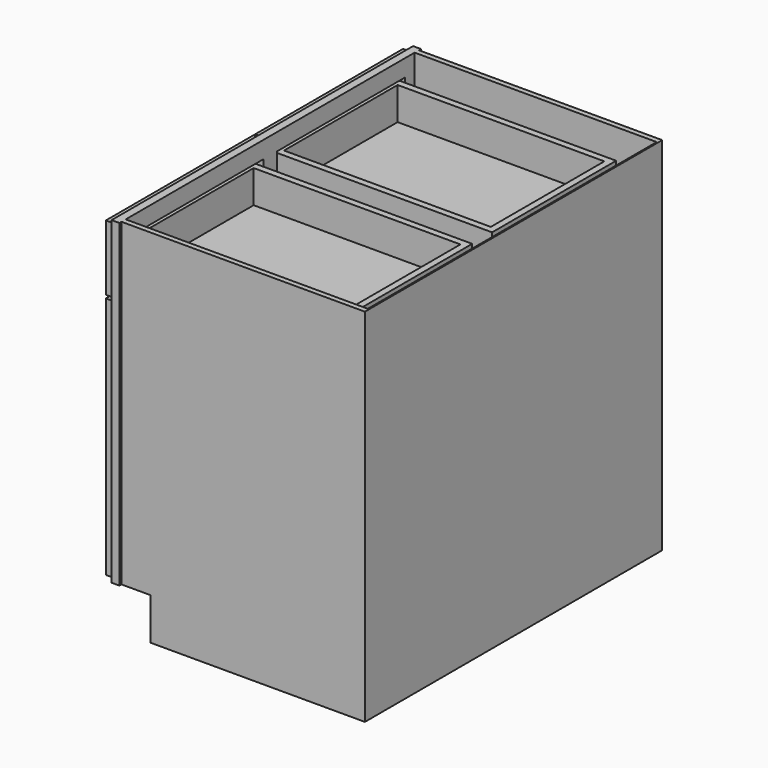
from build123d import *

# Parameters (mm, degrees)
F0_W          = 609.6
F0_H          = 876.3
F1_DEPTH      = 914.4
F2_W          = 88.9
F2_H          = 101.6
F3_DEPTH      = 914.401
F4_W          = 816.9639344262
F4_H          = 692.15
F5_DEPTH      = 19.05
F6_W          = 590.55
F6_H          = 6.35
F7_DEPTH      = 876.301
F8_W          = 587.375
F8_H          = 876.3
F9_DEPTH      = 733.425
F10_W         = 387.8444672131
F10_H         = 41.275
F10_W_2       = 41.275
F10_H_2       = 111.125
F10_H_3       = 539.75
F11_DEPTH     = 19.05
F12_W         = 448.46875
F12_H         = 590.5627
F12_W_2       = 334.16875
F12_H_2       = 476.2627
F13_DEPTH     = 19.05
F14_W         = 6.35
F14_H         = 334.16875
F15_DEPTH     = 476.2627
F16_SIZE      = 3.175
F17_W         = 448.46875
F17_H         = 158.75
F17_W_2       = 334.16875
F17_H_2       = 82.55
F18_DEPTH     = 19.05
F19_W         = 6.35
F19_H         = 334.16875
F20_DEPTH     = 82.55
F21_SIZE      = 3.175
F22_W         = 504.825
F22_H         = 876.3
F23_DEPTH     = 101.6
F24_W         = 376.2375
F24_H         = 95.25
F25_DEPTH     = 533.4
F26_T         = 15.875
F26_T3_DEPTH  = 37.249261314
F26_T5_DEPTH  = 37.249261314
F26_T7_DEPTH  = 37.249261314
F26_T9_DEPTH  = 37.249261314
F26_T11_DEPTH = 36.5125
F26_T13_DEPTH = 365.91875
F26_T15_DEPTH = 114.3
F26_T17_DEPTH = 127
F26_T19_DEPTH = 407.9875
F26_T21_DEPTH = 111.125
F26_T23_DEPTH = 36.5125


# Not quite as in the source:
# - a shell that OpenCascade refuses in one call is made with other operations: the cavity is built on its own and cut out


with BuildPart() as f1:
    # F0 (on Front) → F1 (new body)
    with BuildSketch(Plane.XZ):
        Rectangle(F0_W, F0_H)
    extrude(amount=-F1_DEPTH)

    # F2 (on face) → F3 (cut, through all)
    with BuildSketch(Plane.XZ):
        with Locations((-260.35, -387.35)):
            Rectangle(F2_W, F2_H)
    extrude(amount=-F3_DEPTH, mode=Mode.SUBTRACT)

    # F4 (on face) → F5 (cut)
    with BuildSketch(Plane(origin=(-304.8, 0, 0), x_dir=(0, -1, 0), z_dir=(-1, 0, 0))):
        with Locations((-457.2, 50.8)):
            Rectangle(F4_W, F4_H)
    extrude(amount=-F5_DEPTH, mode=Mode.SUBTRACT)

    # F6 (on face) → F7 (cut, through all)
    with BuildSketch(Plane.XY.offset(438.15)):
        with Locations((9.525, 911.225)):
            Rectangle(F6_W, F6_H)
        with Locations((9.525, 3.175)):
            Rectangle(F6_W, F6_H)
    extrude(amount=-F7_DEPTH, mode=Mode.SUBTRACT)

    # F8 (on face) → F9 (cut, through all)
    with BuildSketch(Plane.XY.offset(438.15)):
        with Locations((7.9375, 457.2)):
            Rectangle(F8_W, F8_H)
    extrude(amount=-F9_DEPTH, mode=Mode.SUBTRACT)

    # F10 (on face) → F11 (join, through all)
    with BuildSketch(Plane(origin=(-304.8, 0, 0), x_dir=(0, -1, 0), z_dir=(-1, 0, 0))):
        with Locations((-671.7597336066, 265.1125)):
            Rectangle(F10_W, F10_H)
        with Locations((-457.2, 341.3125)):
            Rectangle(F10_W_2, F10_H_2)
        with Locations((-457.2, 265.1125)):
            Rectangle(F10_W_2, F10_H)
        with Locations((-242.6402663934, 265.1125)):
            Rectangle(F10_W, F10_H)
        with Locations((-457.2, -25.4)):
            Rectangle(F10_W_2, F10_H_3)
    extrude(amount=-F11_DEPTH)

    # F22 (on face) → F23 (cut)
    with BuildSketch(Plane(origin=(0, 0, -438.15), x_dir=(1, 0, 0), z_dir=(0, 0, -1))):
        with Locations((49.2125, -457.2)):
            Rectangle(F22_W, F22_H)
    extrude(amount=-F23_DEPTH, mode=Mode.SUBTRACT)


with BuildPart() as f13:
    # F12 (on face) → F13 (new body)
    with BuildSketch(Plane(origin=(-304.8, 0, 0), x_dir=(0, -1, 0), z_dir=(-1, 0, 0))):
        with Locations((-683.815625, -33.33115)):
            Rectangle(F12_W, F12_H)
        with Locations((-683.815625, -33.33115)):
            Rectangle(F12_W_2, F12_H_2, mode=Mode.SUBTRACT)
    extrude(amount=F13_DEPTH)

    # F14 (on face) → F15 (join, through all)
    with BuildSketch(Plane.XY.offset(-271.4625)):
        with Locations((-312.7375, 683.815625)):
            Rectangle(F14_W, F14_H)
    extrude(amount=F15_DEPTH)

    # F16
    f16_edges = [f13.edges().sort_by_distance(p)[0] for p in [
        (-323.85, 850.9, -33.33115),
        (-323.85, 683.815625, -271.4625),
        (-323.85, 516.73125, -33.33115),
        (-323.85, 683.815625, 204.8002),
    ]]
    chamfer(f16_edges, length=F16_SIZE)


with BuildPart() as f18:
    # F17 (on face) → F18 (new body)
    with BuildSketch(Plane(origin=(-304.8, 0, 0), x_dir=(0, -1, 0), z_dir=(-1, 0, 0))):
        with Locations((-683.815625, 349.25)):
            Rectangle(F17_W, F17_H)
        with Locations((-683.815625, 349.25)):
            Rectangle(F17_W_2, F17_H_2, mode=Mode.SUBTRACT)
    extrude(amount=F18_DEPTH)

    # F19 (on face) → F20 (join, through all)
    with BuildSketch(Plane.XY.offset(307.975)):
        with Locations((-312.7375, 683.815625)):
            Rectangle(F19_W, F19_H)
    extrude(amount=F20_DEPTH)

    # F21
    f21_edges = [f18.edges().sort_by_distance(p)[0] for p in [
        (-323.85, 683.815625, 307.975),
        (-323.85, 850.9, 349.25),
        (-323.85, 683.815625, 390.525),
        (-323.85, 516.73125, 349.25),
    ]]
    chamfer(f21_edges, length=F21_SIZE)

    # F24 (on face) → F25 (join)
    with BuildSketch(Plane.YZ.offset(-304.8)):
        with Locations((675.48125, 339.725)):
            Rectangle(F24_W, F24_H)
    extrude(amount=F25_DEPTH)

    # F26: shell of thickness 15.875, made by hand


with BuildPart() as f26_core1:
    # F26_t2: copy of F18
    add(f18.part)

    # the walls: a layer under each face that stays
    f26_faces = [f26_core1.faces().sort_by_distance(p)[0] for p in [
        (-323.85, 833.3052083333, 296.3333333333),
        (-322.2625, 683.815625, 306.3875),
        (-322.2625, 515.14375, 349.25),
        (-322.2625, 852.4875, 349.25),
        (-322.2625, 683.815625, 392.1125),
        (-314.325, 683.815625, 428.625),
        (-314.325, 908.05, 349.25),
        (-314.325, 683.815625, 269.875),
        (-314.325, 459.58125, 349.25),
        (-318.29375, 683.815625, 307.975),
        (-318.29375, 516.73125, 349.25),
        (-318.29375, 850.9, 349.25),
        (-318.29375, 683.815625, 390.525),
        (-304.8, 833.3052083333, 402.1666666667),
        (-315.9125, 683.815625, 349.25),
        (-38.1, 863.6, 339.725),
        (-38.1, 675.48125, 292.1),
        (-38.1, 487.3625, 339.725),
        (-307.18125, 516.73125, 349.25),
        (-307.18125, 683.815625, 390.525),
        (-307.18125, 850.9, 349.25),
        (-304.8, 683.815625, 347.6625),
        (228.6, 675.48125, 339.725),
        (-307.18125, 683.815625, 307.975),
        (-309.5625, 683.815625, 349.25),
    ]]
    thicken(f26_faces, amount=-F26_T, mode=Mode.SUBTRACT)

    # F26_s4 → F26_t3 (cut)
    with BuildSketch(Plane(origin=(155.6699811433, 155.6699811433, 155.6699811433), x_dir=(-0.7071067812, 0.7071067812, 0), z_dir=(0.5773502692, 0.5773502692, 0.5773502692))):
        Polygon((592.373762983, 171.5583871468), (584.198137983, 157.6727523289), (576.260637983, 162.2554700906), (576.260637983, 171.420905614), align=None)
    extrude(amount=F26_T3_DEPTH, mode=Mode.SUBTRACT)

    # F26_s6 → F26_t5 (cut)
    with BuildSketch(Plane(origin=(-300.2071021901, 300.20710219, -300.2071021901), x_dir=(0.7071067812, 0.7071067812, 0), z_dir=(0.5773502692, -0.5773502692, 0.5773502692))):
        Polygon((374.6875680546, 729.8915069443), (382.8631930546, 716.0058721263), (390.8006930546, 720.588589888), (390.8006930546, 729.7540254114), align=None)
    extrude(amount=F26_T5_DEPTH, mode=Mode.SUBTRACT)

    # F26_s8 → F26_t7 (cut)
    with BuildSketch(Plane(origin=(-77.1633521901, -77.1633521901, 77.1633521901), x_dir=(-0.7071067812, 0.7071067812, 0), z_dir=(0.5773502692, 0.5773502692, -0.5773502692))):
        Polygon((592.373762983, 398.7644746312), (576.260637983, 398.9019561641), (576.260637983, 408.0673916874), (584.198137983, 412.6501094491), align=None)
    extrude(amount=F26_T7_DEPTH, mode=Mode.SUBTRACT)

    # F26_s10 → F26_t9 (cut)
    with BuildSketch(Plane(origin=(-533.0404355234, 533.0404355234, 533.0404355234), x_dir=(0.7071067812, 0.7071067812, 0), z_dir=(0.5773502692, -0.5773502692, -0.5773502692))):
        Polygon((374.6875680546, -159.5686451663), (390.8006930546, -159.4311636334), (390.8006930546, -150.26572811), (382.8631930546, -145.6830103483), align=None)
    extrude(amount=F26_T9_DEPTH, mode=Mode.SUBTRACT)

    # F26_s12 → F26_t11 (cut)
    with BuildSketch(Plane.YZ.offset(-336.55)):
        Polygon((850.74125, 308.13375), (850.9, 292.1), (866.775, 292.1), (866.775, 307.975), align=None)
        Polygon((516.89, 308.13375), (516.73125, 292.1), (500.85625, 292.1), (500.85625, 307.975), align=None)
        Polygon((516.89, 390.36625), (500.85625, 390.525), (500.85625, 406.4), (516.73125, 406.4), align=None)
        Polygon((850.74125, 390.36625), (866.775, 390.525), (866.775, 406.4), (850.9, 406.4), align=None)
    extrude(amount=F26_T11_DEPTH, mode=Mode.SUBTRACT)

    # F26_s14 → F26_t13 (cut)
    with BuildSketch(Plane.XZ.offset(-866.775)):
        Polygon((-316.07125, 308.13375), (-315.9125, 292.1), (-300.0375, 292.1), (-300.0375, 307.975), align=None)
        Polygon((-316.07125, 390.36625), (-315.9125, 406.4), (-300.0375, 406.4), (-300.0375, 390.525), align=None)
        Polygon((-309.40375, 390.36625), (-309.5625, 406.4), (-325.4375, 406.4), (-325.4375, 390.525), align=None)
        Polygon((-304.95875, 308.13375), (-288.925, 307.975), (-288.925, 292.1), (-304.8, 292.1), align=None)
        Polygon((-309.40375, 308.13375), (-309.5625, 292.1), (-325.4375, 292.1), (-325.4375, 307.975), align=None)
    extrude(amount=F26_T13_DEPTH, mode=Mode.SUBTRACT)

    # F26_s16 → F26_t15 (cut)
    with BuildSketch(Plane.XY.offset(292.1)):
        Polygon((-316.07125, 516.89), (-315.9125, 500.85625), (-300.0375, 500.85625), (-300.0375, 516.73125), align=None)
        Polygon((-316.07125, 850.74125), (-315.9125, 866.775), (-300.0375, 866.775), (-300.0375, 850.9), align=None)
        Polygon((-309.40375, 516.89), (-309.5625, 500.85625), (-325.4375, 500.85625), (-325.4375, 516.73125), align=None)
        Polygon((-309.40375, 850.74125), (-309.5625, 866.775), (-325.4375, 866.775), (-325.4375, 850.9), align=None)
    extrude(amount=F26_T15_DEPTH, mode=Mode.SUBTRACT)

    # F26_s18 → F26_t17 (cut)
    with BuildSketch(Plane.XY.offset(276.225)):
        Polygon((-304.64125, 863.75875), (-320.675, 863.6), (-320.675, 847.725), (-304.8, 847.725), align=None)
        Polygon((-304.64125, 487.20375), (-320.675, 487.3625), (-320.675, 503.2375), (-304.8, 503.2375), align=None)
    extrude(amount=F26_T17_DEPTH, mode=Mode.SUBTRACT)

    # F26_s20 → F26_t19 (cut)
    with BuildSketch(Plane.XZ.offset(-879.475)):
        Polygon((-304.64125, 291.94125), (-320.675, 292.1), (-320.675, 307.975), (-304.8, 307.975), align=None)
    extrude(amount=F26_T19_DEPTH, mode=Mode.SUBTRACT)

    # F26_s22 → F26_t21 (cut)
    with BuildSketch(Plane.XY.offset(292.1)):
        Polygon((-304.95875, 516.89), (-304.8, 500.85625), (-288.925, 500.85625), (-288.925, 516.73125), align=None)
        Polygon((-304.95875, 850.74125), (-304.8, 866.775), (-288.925, 866.775), (-288.925, 850.9), align=None)
    extrude(amount=F26_T21_DEPTH, mode=Mode.SUBTRACT)

    # F26_s24 → F26_t23 (cut)
    with BuildSketch(Plane.YZ.offset(-325.4375)):
        Polygon((516.89, 308.13375), (500.85625, 307.975), (500.85625, 292.1), (516.73125, 292.1), align=None)
        Polygon((516.89, 390.36625), (500.85625, 390.525), (500.85625, 406.4), (516.73125, 406.4), align=None)
        Polygon((850.74125, 390.36625), (850.9, 406.4), (866.775, 406.4), (866.775, 390.525), align=None)
        Polygon((850.74125, 308.13375), (866.775, 307.975), (866.775, 292.1), (850.9, 292.1), align=None)
    extrude(amount=F26_T23_DEPTH, mode=Mode.SUBTRACT)


with BuildPart() as f18_1:
    add(f18.part)

    # what is left inside the walls is the cavity
    f26_cavity = [f26_core1.part.solids().sort_by_distance(p)[0] for p in [
        (45.508333, 675.48125, 308.13375),
    ]]
    add(f26_cavity, mode=Mode.SUBTRACT)


with BuildPart() as f28_1:
    # F28: instance of F18
    add(f18_1.part.mirror(Plane.XZ.offset(-457.2)))


with BuildPart() as f29_1:
    # F29: instance of F13
    add(f13.part.mirror(Plane.XZ.offset(-457.2)))


solid = Compound([f1.part, f13.part, f18_1.part, f28_1.part, f29_1.part])
